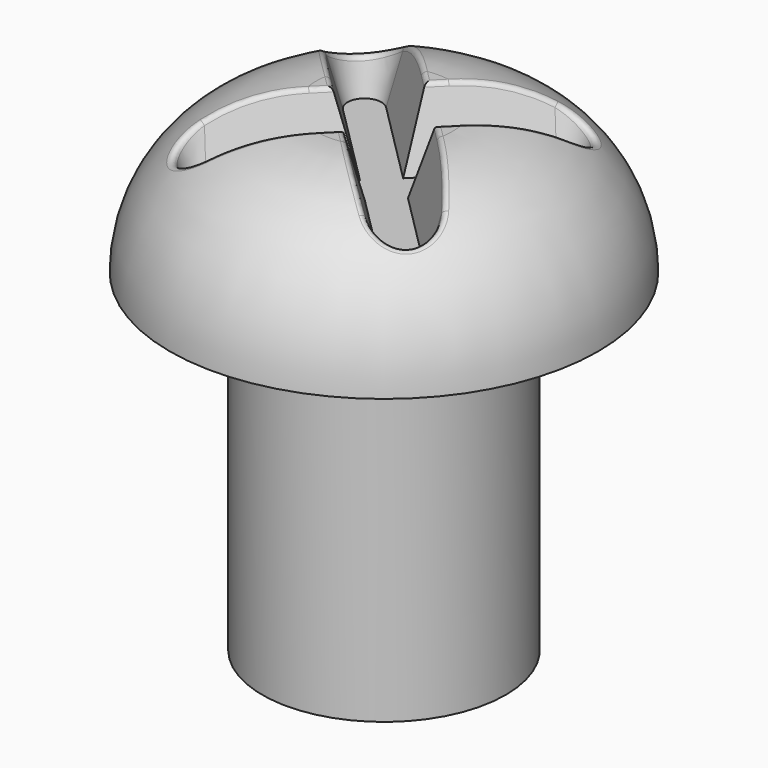
from build123d import *

# Parameters (mm, degrees)
F0_R     = 2.5
F1_DEPTH = 6.83
F2_R     = 4.4
F2_R_2   = 2.5
F3_DEPTH = 3
F4_R     = 2.99999
F6_DEPTH = 1.5
F6_TAPER = 15
F7_R     = 0.1


# Not quite as in the source:
# - a fillet or chamfer is up to 0.001 mm smaller than in the source, because OpenCascade refuses the exact size


with BuildPart() as f1:
    # F0 (on Top) → F1 (new body)
    with BuildSketch(Plane.XY):
        Circle(F0_R)
    extrude(amount=F1_DEPTH)

    # F2 (on face) → F3 (join)
    with BuildSketch(Plane.XY.offset(6.83)):
        Circle(F2_R)
        Circle(F2_R_2, mode=Mode.SUBTRACT)
        Circle(F2_R_2)
    extrude(amount=F3_DEPTH)

    # F4 (radius 3 in the source; OpenCascade refuses exactly that, so slightly less here)
    f4_edges = [f1.edges().sort_by_distance(p)[0] for p in [
        (-4.4, 0, 9.83),
    ]]
    fillet(f4_edges, radius=F4_R)

    # F5 (on face) → F6 (cut)
    with BuildSketch(Plane.XY.offset(9.83)):
        Polygon((-1.0606601718, 0), (-0.5303300859, -0.5303300859), (0, 0), (-0.5303300859, 0.5303300859), align=None)
        with BuildLine():
            Line((0, -1.0606601718), (-0.5303300859, -0.5303300859))
            Line((-0.5303300859, -0.5303300859), (-1.0606601718, 0))
            Line((-1.0606601718, 0), (-2.5303300859, -1.4696699141))
            ThreePointArc((-2.5303300859, -1.4696699141), (-2.5303300859, -2.5303300859), (-1.4696699141, -2.5303300859))
            Line((-1.4696699141, -2.5303300859), (0, -1.0606601718))
        make_face()
        Polygon((0, 0), (-0.5303300859, -0.5303300859), (0, -1.0606601718), (0.5303300859, -0.5303300859), align=None)
        Polygon((-0.5303300859, 0.5303300859), (0, 0), (0.5303300859, 0.5303300859), (0, 1.0606601718), align=None)
        Polygon((0.5303300859, 0.5303300859), (0, 0), (0.5303300859, -0.5303300859), (1.0606601718, 0), align=None)
        with BuildLine():
            Line((-2.5303300859, 1.4696699141), (-1.0606601718, 0))
            Line((-1.0606601718, 0), (-0.5303300859, 0.5303300859))
            Line((-0.5303300859, 0.5303300859), (0, 1.0606601718))
            Line((0, 1.0606601718), (-1.4696699141, 2.5303300859))
            ThreePointArc((-1.4696699141, 2.5303300859), (-2.5303300859, 2.5303300859), (-2.5303300859, 1.4696699141))
        make_face()
        with BuildLine():
            Line((0.5303300859, -0.5303300859), (0, -1.0606601718))
            Line((0, -1.0606601718), (1.4696699141, -2.5303300859))
            ThreePointArc((1.4696699141, -2.5303300859), (2.5303300859, -2.5303300859), (2.5303300859, -1.4696699141))
            Line((2.5303300859, -1.4696699141), (1.0606601718, 0))
            Line((1.0606601718, 0), (0.5303300859, -0.5303300859))
        make_face()
        with BuildLine():
            Line((0, 1.0606601718), (0.5303300859, 0.5303300859))
            Line((0.5303300859, 0.5303300859), (1.0606601718, 0))
            Line((1.0606601718, 0), (2.5303300859, 1.4696699141))
            ThreePointArc((2.5303300859, 1.4696699141), (2.5303300859, 2.5303300859), (1.4696699141, 2.5303300859))
            Line((1.4696699141, 2.5303300859), (0, 1.0606601718))
        make_face()
    extrude(amount=-F6_DEPTH, taper=F6_TAPER, mode=Mode.SUBTRACT)

    # F7
    f7_edges = [f1.edges().sort_by_distance(p)[0] for p in [
        (0.925446, -1.949244, 9.732721),
        (1.949244, 0.925446, 9.732721),
        (0.925446, 1.949244, 9.732721),
        (-0.925446, 1.949244, 9.732721),
        (-1.949244, -0.925446, 9.732721),
    ]]
    fillet(f7_edges, radius=F7_R)


solid = f1.part
